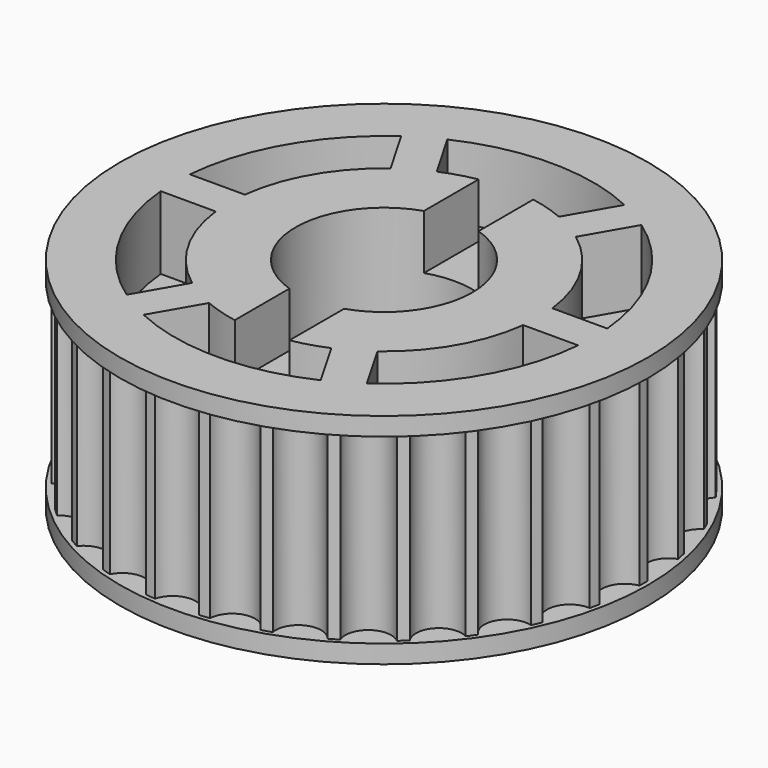
from build123d import *

# Parameters (mm, degrees)
F0_R            = 14.5
F1_DEPTH        = 1
F2_R            = 14.5
F3_DEPTH        = 11
F4_R            = 1.25
F5_DEPTH        = 10
F5_COPIES_COUNT = 30
F6_R            = 14.5
F6_R_2          = 14.25
F7_DEPTH        = 10
F9_DEPTH        = 4
F9_COPIES_COUNT = 3
F10_R           = 4.85
F11_DEPTH       = 12.001
F12_W           = 3
F12_H           = 18.4240331947
F13_DEPTH       = 3


# Not quite as in the source:
# - a pattern or mirror of a feature is missing from the dataset's text; its kind, count and spacing are read off the source's solid


with BuildPart() as f1:
    # F0 (on Top) → F1 (new body)
    with BuildSketch(Plane.XY):
        Circle(F0_R)
    extrude(amount=F1_DEPTH)


with BuildPart() as f3:
    # F2 (on face) → F3 (new body)
    with BuildSketch(Plane.XY.offset(1)):
        Circle(F2_R)
    extrude(amount=F3_DEPTH)

    # F4 (on face) → F5 (cut)
    with BuildSketch(Plane(origin=(0, 0, 1), x_dir=(1, 0, 0), z_dir=(0, 0, -1))):
        with Locations((0, -14.5)):
            Circle(F4_R)
    f5 = extrude(amount=-F5_DEPTH, mode=Mode.SUBTRACT)

    # F5_copies: F5 ×30 about axis
    f5_copies_axis = Axis((0, 0, 0), (0, 0, 1))
    for i in range(1, F5_COPIES_COUNT):
        add(f5.rotate(f5_copies_axis, i * 360 / F5_COPIES_COUNT), mode=Mode.SUBTRACT)

    # F6 (on face) → F7 (cut)
    with BuildSketch(Plane(origin=(0, 0, 1), x_dir=(1, 0, 0), z_dir=(0, 0, -1))):
        Circle(F6_R)
        Circle(F6_R_2, mode=Mode.SUBTRACT)
    extrude(amount=-F7_DEPTH, mode=Mode.SUBTRACT)

    # F8 (on face) → F9 (cut)
    with BuildSketch(Plane.XY.offset(12)):
        with BuildLine():
            Line((-5.0865111578, 6.8100957586), (-6.5942450225, 9.4215674165))
            ThreePointArc((-6.5942450225, 9.4215674165), (-9.9592921435, 5.75), (-11.4564392374, 1))
            Line((-11.4564392374, 1), (-8.4409715081, 1))
            ThreePointArc((-8.4409715081, 1), (-7.3612159322, 4.25), (-5.0865111578, 6.8100957586))
        make_face()
    f9 = extrude(amount=-F9_DEPTH, mode=Mode.SUBTRACT)

    # F9_copies: F9 ×3 about axis
    f9_copies_axis = Axis((0, 0, 0), (0, 0, 1))
    for i in range(1, F9_COPIES_COUNT):
        add(f9.rotate(f9_copies_axis, i * 360 / F9_COPIES_COUNT), mode=Mode.SUBTRACT)

    # F9_copies1: F9 across plane
    add(f9.mirror(Plane(origin=(0, 0, 0), x_dir=(0.5, 0.8660254038, 0), z_dir=(0.8660254038, -0.5, 0))), mode=Mode.SUBTRACT)

    # F9_copies2: F9 across plane
    add(f9.mirror(Plane(origin=(0, 0, 0), x_dir=(0, 0, -1), z_dir=(0, -1, 0))), mode=Mode.SUBTRACT)

    # F9_copies3: F9 across plane
    add(f9.mirror(Plane(origin=(0, 0, 0), x_dir=(-0.5, 0.8660254038, 0), z_dir=(0.8660254038, 0.5, 0))), mode=Mode.SUBTRACT)


with BuildPart() as f11_tool:
    # F10 (on face) → F11 (new body, through all)
    with BuildSketch(Plane.XY.offset(12)):
        Circle(F10_R)
    extrude(amount=-F11_DEPTH)


with BuildPart() as f1_1:
    add(f1.part)

    # F11: cut by f11_tool
    add(f11_tool.part, mode=Mode.SUBTRACT)


with BuildPart() as f3_1:
    add(f3.part)

    # F11: cut by f11_tool
    add(f11_tool.part, mode=Mode.SUBTRACT)

    # F12 (on face) → F13 (cut)
    with BuildSketch(Plane.XY.offset(12)):
        Rectangle(F12_W, F12_H)
    extrude(amount=-F13_DEPTH, mode=Mode.SUBTRACT)


solid = Compound([f1_1.part, f3_1.part])
